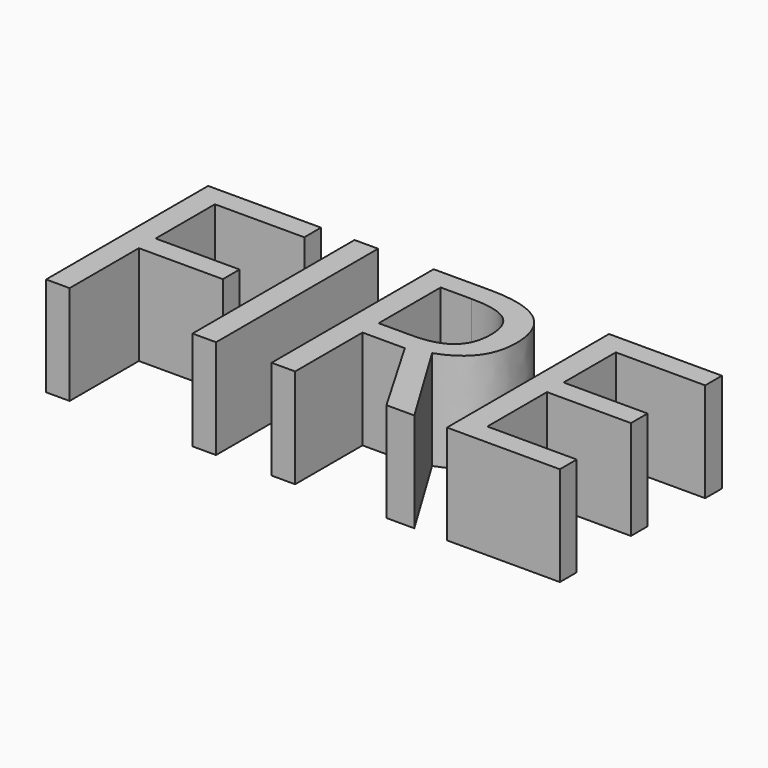
from build123d import *

# Parameters (mm, degrees)
F0_TEXT_SIZE = 72.5325973084
F1_DEPTH     = 25.4


# Not quite as in the source:
# - Text() gives the source's letters only with a copy of the font that has no kerning and outlines rounded to 1/6400 em; it was checked with that copy


with BuildPart() as f1:
    # F0 (on Top) → F1 (new body)
    with BuildSketch(Plane.XY):
        with Locations((-113.2573336363, -35.729251802)):
            Text('FIRE', F0_TEXT_SIZE, font='Open Sans', text_align=(TextAlign.LEFT, TextAlign.BOTTOM))
    extrude(amount=F1_DEPTH)


solid = f1.part
